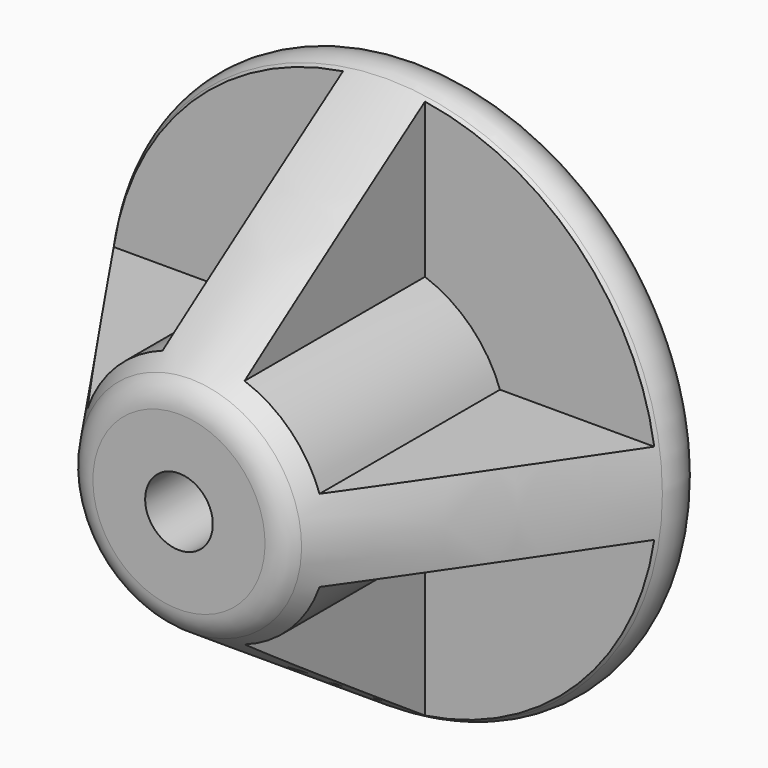
from build123d import *

# Parameters (mm, degrees)
F3_D     = 6.6
F5_D     = 17.4
F5_DEPTH = 12
F5_TIP   = 5.2274873855
F6_D     = 19
F6_DEPTH = 5
F6_TIP   = 5.7081758808
F7_DEPTH = 25
F8_R     = 3


with BuildPart() as f1:
    # F0 (on Right) → F1 (revolve)
    with BuildSketch(Plane.YZ):
        Polygon((-30, 0), (0, 0), (0, 30), (-30, 10), align=None)
    revolve(axis=Axis((0, -15, 0), (0, -1, 0)))

    # F3 (through all)
    with Locations(Plane.XZ.offset(30)):
        with Locations((0, 0)):
            Hole(F3_D / 2)

    # F5
    with Locations(Plane(origin=(0, 0, 0), x_dir=(-1, 0, 0), z_dir=(0, 1, 0))):
        with Locations((0, 0)):
            Hole(F5_D / 2, depth=F5_DEPTH)
            with Locations((0, 0, -(F5_DEPTH + F5_TIP / 2))):  # 118° drill point
                Cone(0, F5_D / 2, F5_TIP, mode=Mode.SUBTRACT)

    # F6
    with Locations(Plane(origin=(0, 0, 0), x_dir=(-1, 0, 0), z_dir=(0, 1, 0))):
        with Locations((0, 0)):
            Hole(F6_D / 2, depth=F6_DEPTH)
            with Locations((0, 0, -(F6_DEPTH + F6_TIP / 2))):  # 118° drill point
                Cone(0, F6_D / 2, F6_TIP, mode=Mode.SUBTRACT)

    # F2 (on face) → F7 (cut)
    with BuildSketch(Plane.XZ.offset(30)):
        with BuildLine():
            ThreePointArc((11.313708499, -4), (8.4852813742, -8.4852813742), (4, -11.313708499))
            Line((4, -11.313708499), (4, -27.313708499))
            ThreePointArc((4, -27.313708499), (19.5197165959, -19.5197165959), (27.313708499, -4))
            Line((27.313708499, -4), (11.313708499, -4))
        make_face()
        with BuildLine():
            Line((11.313708499, 4), (27.313708499, 4))
            ThreePointArc((27.313708499, 4), (19.5197165959, 19.5197165959), (4, 27.313708499))
            Line((4, 27.313708499), (4, 11.313708499))
            ThreePointArc((4, 11.313708499), (8.4852813742, 8.4852813742), (11.313708499, 4))
        make_face()
        with BuildLine():
            Line((-4, 11.313708499), (-4, 27.313708499))
            ThreePointArc((-4, 27.313708499), (-19.5197165959, 19.5197165959), (-27.313708499, 4))
            Line((-27.313708499, 4), (-11.313708499, 4))
            ThreePointArc((-11.313708499, 4), (-8.4852813742, 8.4852813742), (-4, 11.313708499))
        make_face()
        with BuildLine():
            Line((-11.313708499, -4), (-27.313708499, -4))
            ThreePointArc((-27.313708499, -4), (-19.5197165959, -19.5197165959), (-4, -27.313708499))
            Line((-4, -27.313708499), (-4, -11.313708499))
            ThreePointArc((-4, -11.313708499), (-8.4852813742, -8.4852813742), (-11.313708499, -4))
        make_face()
    extrude(amount=-F7_DEPTH, mode=Mode.SUBTRACT)

    # F8
    f8_edges = [f1.edges().sort_by_distance(p)[0] for p in [
        (0, 0, -30),
        (0, -30, -10),
    ]]
    fillet(f8_edges, radius=F8_R)


solid = f1.part
